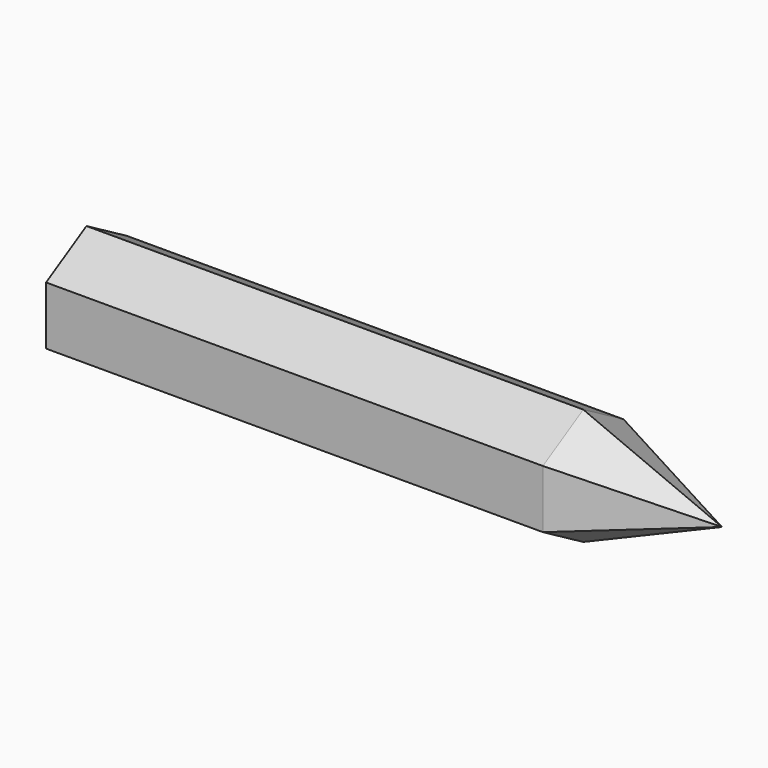
from build123d import *

# Parameters (mm, degrees)
F1_DEPTH = 203.2


# Not quite as in the source:
# - an extrude whose draft closes it to a point is written as a loft to that point


with BuildPart() as f1:
    # F0 (on Right) → F1 (new body)
    with BuildSketch(Plane.YZ):
        Polygon((20.6375, 11.9150661804), (0, 23.8301323608), (-20.6375, 11.9150661804), (-20.6375, -11.9150661804), (0, -23.8301323608), (20.6375, -11.9150661804), align=None)
    extrude(amount=F1_DEPTH)


with BuildPart() as f3:
    # F2 (on face) → F3 section 0
    with BuildSketch(Plane.YZ.offset(203.2), mode=Mode.PRIVATE) as f3_s0:
        Polygon((20.6375, 11.9150661804), (0, 23.8301323608), (-20.6375, 11.9150661804), (-20.6375, -11.9150661804), (0, -23.8301323608), (20.6375, -11.9150661804), align=None)
    loft([f3_s0.sketch, Vertex(259.901065244, 0, 0)], ruled=True)


solid = Compound([f1.part, f3.part])
